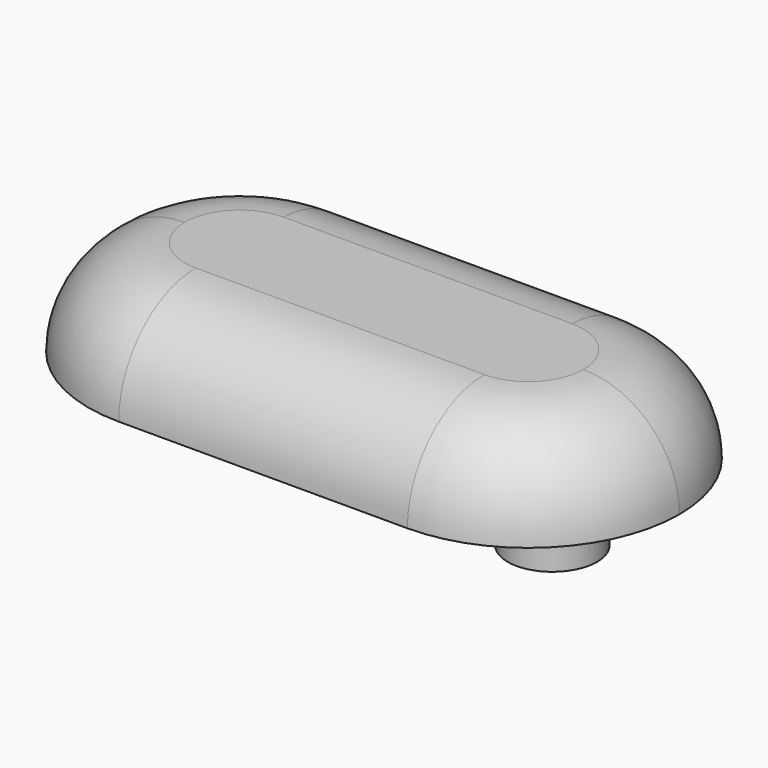
from build123d import *

# Parameters (mm, degrees)
F0_R     = 5.25
F0_R_2   = 3.25
F0_R_3   = 1.75
F1_DEPTH = 7
F2_R     = 6.99999
F3_DEPTH = 5
F4_DEPTH = 0.2
F5_SIZE  = 0.5
F6_R     = 2.75
F6_R_2   = 1.75
F7_DEPTH = 0.5


# Not quite as in the source:
# - a fillet or chamfer is up to 0.001 mm smaller than in the source, because OpenCascade refuses the exact size
# - a feature names something its author has since deleted; it is built from what else it names


with BuildPart() as f1:
    # F0 (on Top) → F1 (new body)
    with BuildSketch(Plane.XY):
        with BuildLine():
            Line((10.5, 11), (-10.5, 11))
            ThreePointArc((-10.5, 11), (-18.2781745931, 7.7781745931), (-21.5, 0))
            ThreePointArc((-21.5, 0), (-18.2781745931, -7.7781745931), (-10.5, -11))
            Line((-10.5, -11), (10.5, -11))
            ThreePointArc((10.5, -11), (18.2781745931, -7.7781745931), (21.5, 0))
            ThreePointArc((21.5, 0), (18.2781745931, 7.7781745931), (10.5, 11))
        make_face()
        with Locations((-12.25, 0)):
            Circle(F0_R, mode=Mode.SUBTRACT)
        with Locations((12.25, 0)):
            Circle(F0_R, mode=Mode.SUBTRACT)
        with Locations((-12.25, 0)):
            Circle(F0_R)
        with Locations((-12.25, 0)):
            Circle(F0_R_2, mode=Mode.SUBTRACT)
        with Locations((12.25, 0)):
            Circle(F0_R)
        with Locations((12.25, 0)):
            Circle(F0_R_2, mode=Mode.SUBTRACT)
        with Locations((12.25, 0)):
            Circle(F0_R_2)
        with Locations((12.25, 0)):
            Circle(F0_R_3, mode=Mode.SUBTRACT)
        with Locations((-12.25, 0)):
            Circle(F0_R_2)
        with Locations((-12.25, 0)):
            Circle(F0_R_3, mode=Mode.SUBTRACT)
        with Locations((-12.25, 0)):
            Circle(F0_R_3)
        with Locations((12.25, 0)):
            Circle(F0_R_3)
    extrude(amount=F1_DEPTH)

    # F2 (radius 7 in the source; OpenCascade refuses exactly that, so slightly less here)
    f2_edges = [f1.edges().sort_by_distance(p)[0] for p in [
        (0, 11, 7),
    ]]
    fillet(f2_edges, radius=F2_R)

    # F0 (on Top) → F3 (join)
    with BuildSketch(Plane.XY):
        with Locations((12.25, 0)):
            Circle(F0_R_2)
        with Locations((12.25, 0)):
            Circle(F0_R_3, mode=Mode.SUBTRACT)
        with Locations((-12.25, 0)):
            Circle(F0_R_2)
        with Locations((-12.25, 0)):
            Circle(F0_R_3, mode=Mode.SUBTRACT)
    extrude(amount=-F3_DEPTH)

    # F0 (on Top) → F4 (cut)
    with BuildSketch(Plane.XY):
        with Locations((-12.25, 0)):
            Circle(F0_R)
        with Locations((-12.25, 0)):
            Circle(F0_R_2, mode=Mode.SUBTRACT)
        with Locations((12.25, 0)):
            Circle(F0_R)
        with Locations((12.25, 0)):
            Circle(F0_R_2, mode=Mode.SUBTRACT)
    extrude(amount=F4_DEPTH, mode=Mode.SUBTRACT)

    # F5
    f5_edges = [f1.edges().sort_by_distance(p)[0] for p in [
        (-15.5, 0, 0.2),
        (9, 0, 0.2),
    ]]
    chamfer(f5_edges, length=F5_SIZE)

    # F6 (on face) → F7 (cut)
    with BuildSketch(Plane(origin=(0, 0, -5), x_dir=(1, 0, 0), z_dir=(0, 0, -1))):
        with Locations((-12.25, 0)):
            Circle(F6_R)
        with Locations((-12.25, 0)):
            Circle(F6_R_2, mode=Mode.SUBTRACT)
        with Locations((12.25, 0)):
            Circle(F6_R)
    extrude(amount=-F7_DEPTH, mode=Mode.SUBTRACT)


solid = f1.part
